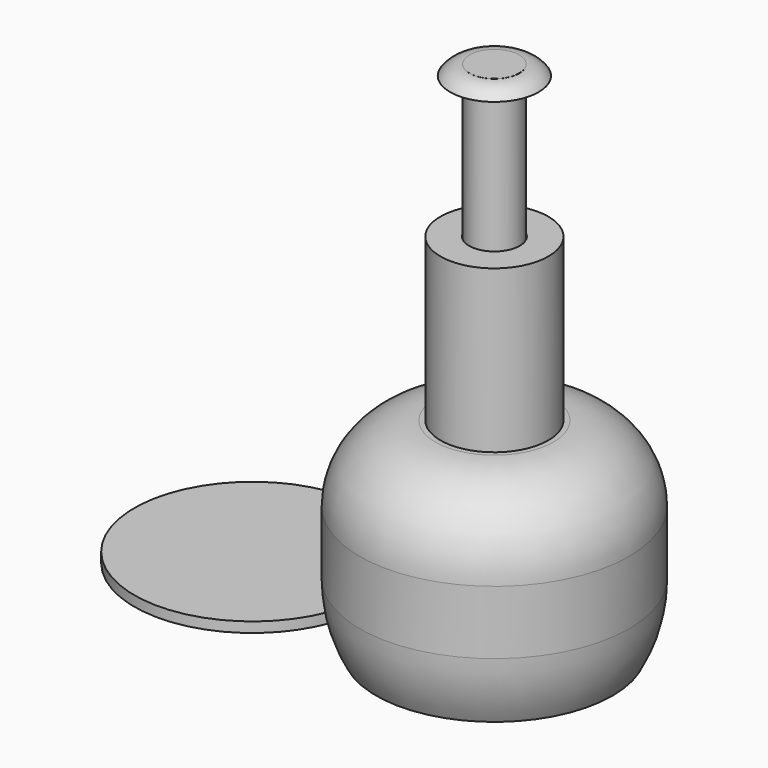
from build123d import *

# Parameters (mm, degrees)
F0_R           = 12.7
F1_DEPTH       = 38.1
F2_R           = 5.9627881531
F3_DEPTH       = 38.101
F4_R           = 31.7446048685
F5_DEPTH       = 23
F6_DEPTH       = 25
F7_R           = 27.8082327549
F8_DEPTH       = 41
F9_DEPTH       = 49
F10_R          = 17.8651803616
F13_DEPTH      = 38.3
F14_DEPTH      = 7.9
F15_W          = 12.8781338312
F15_H          = 29.2036004663
F16_DEPTH      = 3.3
F17_W          = 1.7227437347
F17_H          = 12.1852611192
F18_DEPTH      = 3.1
F19_R          = 27.8
F20_DEPTH      = 48.1
F21_DEPTH      = 45.7
F23_DEPTH      = 0.6
F24_R          = 5.8374914011
F25_DEPTH      = 27.1
F26_DEPTH      = 71.4
F27_R          = 10.4165090819
F27_R_2        = 5.8374914011
F28_DEPTH      = 2.4
F29_DEPTH      = 2.6
F30_DEPTH      = 3.3
F31_DEPTH      = 1.2
F32_T4_DEPTH   = 20.0314551969
F32_2_T1_DEPTH = 17.4227077627
F33_SIZE       = 5.835
F35_DEPTH      = 0.18
F36_T1_DEPTH   = 13.8587724822
F36_T3_DEPTH   = 8.1698239296
F36_T5_DEPTH   = 21.2291069713
F36_T7_DEPTH   = 7.7223795322
F36_T9_DEPTH   = 14.3062168796


# Not quite as in the source:
# - a fillet or chamfer that OpenCascade refuses, or shapes differently, is made with other operations: its cross-section is extruded or revolved along the edge and cut away or added


with BuildPart() as f1:
    # F0 (on Top) → F1 (new body)
    with BuildSketch(Plane.XY):
        Circle(F0_R)
    extrude(amount=F1_DEPTH)

    # F2 (on face) → F3 (cut, through all)
    with BuildSketch(Plane.XY.offset(38.1)):
        Circle(F2_R)
    extrude(amount=-F3_DEPTH, mode=Mode.SUBTRACT)

    # F4 (on Top) → F5 (join)
    with BuildSketch(Plane.XY):
        Circle(F4_R)
    extrude(amount=-F5_DEPTH)

    # F6 (add): a face of the model
    f6_faces = [f1.faces().sort_by_distance(p)[0] for p in [
        (0, 0, -23),
    ]]
    extrude(f6_faces, amount=F6_DEPTH)

    # F7 (on face) → F8 (cut)
    with BuildSketch(Plane(origin=(0, 0, -48), x_dir=(1, 0, 0), z_dir=(0, 0, -1))):
        Circle(F7_R)
    extrude(amount=-F8_DEPTH, mode=Mode.SUBTRACT)

    # F9 (cut): a face of the model
    f9_faces = [f1.faces().sort_by_distance(p)[0] for p in [
        (0, 0, 0),
    ]]
    extrude(f9_faces, amount=-F9_DEPTH, mode=Mode.SUBTRACT)

    # F10
    f10_edges = [f1.edges().sort_by_distance(p)[0] for p in [
        (-31.744605, 0, 0),
    ]]
    fillet(f10_edges, radius=F10_R)

    # F11: fillet of radius 31.1433549546 on 1 edges, made by hand

    # F11_s1 → F11_t2 (revolve, cut)
    with BuildSketch(Plane.XZ):
        with BuildLine():
            ThreePointArc((31.7446048685, -32.8445177405), (30.7444521466, -40.6736886407), (27.8082327549, -48))
            Line((27.8082327549, -48), (28.3523724117, -48.3031096452))
            ThreePointArc((28.3523724117, -48.3031096452), (29.7764188117, -48.6228670991), (31.7446048685, -48.6228670991))
            Line((31.7446048685, -48.6228670991), (32.3674719676, -48))
            Line((32.3674719676, -48), (32.3674719676, -32.8445177405))
            Line((32.3674719676, -32.8445177405), (31.7446048685, -32.8445177405))
        make_face()
    revolve(axis=Axis((0, 0, -48), (0, 0, 1)), mode=Mode.SUBTRACT)

    # F12 (on face) → F13 (join)
    with BuildSketch(Plane(origin=(0, 0, -7), x_dir=(1, 0, 0), z_dir=(0, 0, -1))):
        with BuildLine():
            ThreePointArc((-27.3590203134, 4.9781338312), (-27.6957019569, 2.4991802785), (-27.8082327549, 0))
            Line((-27.8082327549, 0), (-23.2980027795, 0))
            Line((-23.2980027795, 0), (-23.2980027795, 4.9781338312))
            Line((-23.2980027795, 4.9781338312), (-27.3590203134, 4.9781338312))
        make_face()
    extrude(amount=F13_DEPTH)

    # F14 (add): a face of the model
    f14_faces = [f1.faces().sort_by_distance(p)[0] for p in [
        (-25.5531177672, 0, -26.15),
    ]]
    extrude(f14_faces, amount=F14_DEPTH)

    # F15 (on face) → F16 (cut)
    with BuildSketch(Plane.YZ.offset(-23.2980027795)):
        with Locations((1.4609330844, -21.6018002331)):
            Rectangle(F15_W, F15_H)
    extrude(amount=-F16_DEPTH, mode=Mode.SUBTRACT)

    # F17 (on face) → F18 (join)
    with BuildSketch(Plane(origin=(0, 0, -45.3), x_dir=(1, 0, 0), z_dir=(0, 0, -1))):
        with Locations((-25.5140950903, -1.4316115994)):
            Rectangle(F17_W, F17_H)
    extrude(amount=F18_DEPTH)

    # F31 (add): a face of the model
    f31_faces = [f1.faces().sort_by_distance(p)[0] for p in [
        (-24.652723223, 1.4316115994, -46.85),
    ]]
    extrude(f31_faces, amount=F31_DEPTH)

    # F32: fillet of radius 3.1384776311 on 1 edges, made by hand


with BuildPart() as f20:
    # F19 (on Top) → F20 (new body)
    with BuildSketch(Plane.XY):
        with Locations((-56.9376163185, 0)):
            Circle(F19_R)
    extrude(amount=-F20_DEPTH)

    # F21 (cut): a face of the model
    f21_faces = [f20.faces().sort_by_distance(p)[0] for p in [
        (-56.9376163185, 0, 0),
    ]]
    extrude(f21_faces, amount=-F21_DEPTH, mode=Mode.SUBTRACT)

    # F22 (on face) → F23 (join)
    with BuildSketch(Plane(origin=(0, 0, -48.1), x_dir=(1, 0, 0), z_dir=(0, 0, -1))):
        with BuildLine():
            ThreePointArc((-29.1376163185, 0), (-29.1680566948, 1.3005992115), (-29.2593111608, 2.5983501691))
            Line((-29.2593111608, 2.5983501691), (-37.0483733714, 2.5983501691))
            Line((-37.0483733714, 2.5983501691), (-37.0483733714, -5.5964472704))
            Line((-37.0483733714, -5.5964472704), (-29.7067555544, -5.5964472704))
            ThreePointArc((-29.7067555544, -5.5964472704), (-29.2802671212, -2.8126562854), (-29.1376163185, 0))
        make_face()
        with BuildLine():
            Line((-28.0540864915, -5.5964472704), (-28.0540864915, 2.5983501691))
            Line((-28.0540864915, 2.5983501691), (-29.2593111608, 2.5983501691))
            ThreePointArc((-29.2593111608, 2.5983501691), (-29.1680566948, 1.3005992115), (-29.1376163185, 0))
            ThreePointArc((-29.1376163185, 0), (-29.2802671212, -2.8126562854), (-29.7067555544, -5.5964472704))
            Line((-29.7067555544, -5.5964472704), (-28.0540864915, -5.5964472704))
        make_face()
    extrude(amount=F23_DEPTH)


with BuildPart() as f25:
    # F24 (on Top) → F25 (new body)
    with BuildSketch(Plane.XY):
        Circle(F24_R)
    extrude(amount=-F25_DEPTH)

    # F26 (add): a face of the model
    f26_faces = [f25.faces().sort_by_distance(p)[0] for p in [
        (0, 0, 0),
    ]]
    extrude(f26_faces, amount=F26_DEPTH)


with BuildPart() as f28:
    # F27 (on face) → F28 (new body)
    with BuildSketch(Plane.XY.offset(71.4)):
        Circle(F27_R)
        Circle(F27_R_2, mode=Mode.SUBTRACT)
    extrude(amount=F28_DEPTH)

    # F34: fillet of radius 5.5526911935 on 1 edges, made by hand

    # F34_s1 → F34_t2 (revolve, cut)
    with BuildSketch(Plane.XZ):
        with BuildLine():
            ThreePointArc((10.4165090819, 71.4), (8.426955147, 73.1635217858), (5.8456319529, 73.8))
            Line((5.8456319529, 73.8), (10.4165090819, 73.8))
            Line((10.4165090819, 73.8), (10.4165090819, 71.4))
        make_face()
    revolve(axis=Axis((0, 0, 73.8), (0, 0, 1)), mode=Mode.SUBTRACT)


with BuildPart() as f29:
    # F29 (new): a face of the model
    f29_faces = [f25.part.faces().sort_by_distance(p)[0] for p in [
        (0, 0, 71.4),
    ]]
    extrude(f29_faces, amount=F29_DEPTH)

    # F35 (cut): a face of the model
    f35_faces = [f29.faces().sort_by_distance(p)[0] for p in [
        (0, 0, 74),
    ]]
    extrude(f35_faces, amount=-F35_DEPTH, mode=Mode.SUBTRACT)


with BuildPart() as f30:
    # F30 (new): a face of the model
    f30_faces = [f20.part.faces().sort_by_distance(p)[0] for p in [
        (-28.0540864915, 1.4990485506, -48.4),
    ]]
    extrude(f30_faces, amount=F30_DEPTH)

    # F32#2: fillet of radius 3.1384776311 on 1 edges, made by hand

    # F32_2_s2 → F32_2_t1 (cut)
    with BuildSketch(Plane.XZ.offset(-10.210402432)):
        with BuildLine():
            ThreePointArc((-26.5996685561, -48.7), (-25.6293370203, -48.5462331676), (-24.7540864915, -48.1))
            Line((-24.7540864915, -48.1), (-24.7540864915, -48.7))
            Line((-24.7540864915, -48.7), (-26.5996685561, -48.7))
        make_face()
    extrude(amount=F32_2_T1_DEPTH, mode=Mode.SUBTRACT)


with BuildPart() as f32_tool2:
    # F32_s3 → F32_t4 (new body)
    with BuildSketch(Plane.XZ.offset(-7.524242159)):
        with BuildLine():
            ThreePointArc((-26.5912008541, -48.4), (-24.3719620385, -47.4807611845), (-23.452723223, -45.2615223689))
            Line((-23.452723223, -45.2615223689), (-23.452723223, -48.4))
            Line((-23.452723223, -48.4), (-26.5912008541, -48.4))
        make_face()
    extrude(amount=F32_T4_DEPTH)

    split(bisect_by=Plane.XY.offset(-45.3), keep=Keep.BOTTOM)

    split(bisect_by=Plane.XZ.offset(4.9781338312), keep=Keep.BOTTOM)


with BuildPart() as f1_1:
    add(f1.part)

    # F32_t1: cut F32_tool2
    add(f32_tool2.part, mode=Mode.SUBTRACT)


with BuildPart() as f25_1:
    add(f25.part)

    # F33
    f33_edges = [f25_1.edges().sort_by_distance(p)[0] for p in [
        (-5.837491, 0, -27.1),
    ]]
    chamfer(f33_edges, length=F33_SIZE)


with BuildPart() as f20_1:
    add(f20.part)

    # F36: fillet of radius 5.9631074991 on 3 edges, made by hand

    # F36_s2 → F36_t1 (cut)
    with BuildSketch(Plane.YZ.offset(-43.5655281373)):
        with BuildLine():
            ThreePointArc((5.5964472704, -48.1), (4.3270950835, -48.5480643961), (2.989585364, -48.7))
            Line((2.989585364, -48.7), (5.5964472704, -48.7))
            Line((5.5964472704, -48.7), (5.5964472704, -48.1))
        make_face()
    extrude(amount=F36_T1_DEPTH, mode=Mode.SUBTRACT)

    # F36_s4 → F36_t3 (cut)
    with BuildSketch(Plane.YZ.offset(-29.7067556551)):
        with BuildLine():
            ThreePointArc((5.5964472704, -48.1), (4.3270950835, -48.5480643961), (2.989585364, -48.7))
            Line((2.989585364, -48.7), (5.5964472704, -48.7))
            Line((5.5964472704, -48.7), (5.5964472704, -48.1))
        make_face()
    extrude(amount=F36_T3_DEPTH, mode=Mode.SUBTRACT)

    # F36_s6 → F36_t5 (cut)
    with BuildSketch(Plane.XZ.offset(-12.1136020363)):
        with BuildLine():
            ThreePointArc((-37.0483733714, -48.1), (-35.7790211845, -48.5480643961), (-34.441511465, -48.7))
            Line((-34.441511465, -48.7), (-37.0483733714, -48.7))
            Line((-37.0483733714, -48.7), (-37.0483733714, -48.1))
        make_face()
    extrude(amount=F36_T5_DEPTH, mode=Mode.SUBTRACT)

    # F36_s8 → F36_t7 (cut)
    with BuildSketch(Plane.YZ.offset(-29.2593112577)):
        with BuildLine():
            ThreePointArc((-2.5983501691, -48.1), (-1.3289979823, -48.5480643961), (0.0085117372, -48.7))
            Line((0.0085117372, -48.7), (-2.5983501691, -48.7))
            Line((-2.5983501691, -48.7), (-2.5983501691, -48.1))
        make_face()
    extrude(amount=F36_T7_DEPTH, mode=Mode.SUBTRACT)

    # F36_s10 → F36_t9 (cut)
    with BuildSketch(Plane.YZ.offset(-43.5655281373)):
        with BuildLine():
            ThreePointArc((-2.5983501691, -48.1), (-1.3289979823, -48.5480643961), (0.0085117372, -48.7))
            Line((0.0085117372, -48.7), (-2.5983501691, -48.7))
            Line((-2.5983501691, -48.7), (-2.5983501691, -48.1))
        make_face()
    extrude(amount=F36_T9_DEPTH, mode=Mode.SUBTRACT)


solid = Compound([f28.part, f29.part, f30.part, f1_1.part, f25_1.part, f20_1.part])
